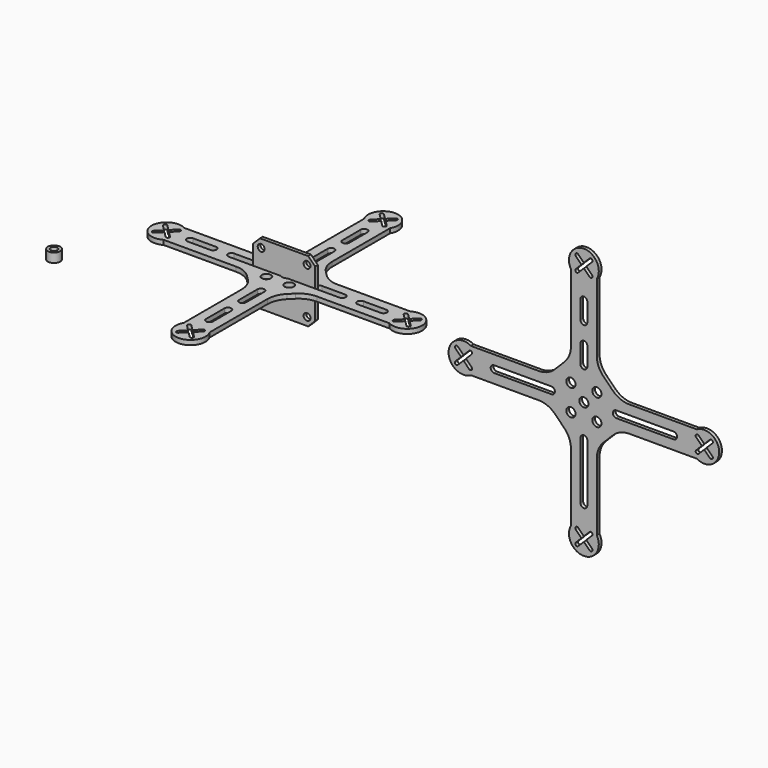
from build123d import *

# Parameters (mm, degrees)
F0_R     = 1.5
F1_DEPTH = 1.5
F0_R_2   = 2
F2_R     = 2
F3_DEPTH = 2
F2_R_2   = 2.7
F2_R_3   = 1.5
F4_DEPTH = 4


# Not quite as in the source:
# - ends of sketch curves that miss each other by under 0.0002 mm in the source are joined


with BuildPart() as f1:
    # F0 (on Front) → F1 (new body)
    with BuildSketch(Plane.XZ):
        Polygon((-10.5, 13.5), (-13.5, 10.5), (-13.5, -10.5), (-10.5, -13.5), (10.5, -13.5), (13.5, -10.5), (13.5, 10.5), (10.5, 13.5), align=None)
        with Locations((-10, -10)):
            Circle(F0_R, mode=Mode.SUBTRACT)
        with Locations((10, -10)):
            Circle(F0_R, mode=Mode.SUBTRACT)
        with Locations((-10, 10)):
            Circle(F0_R, mode=Mode.SUBTRACT)
        with Locations((10, 10)):
            Circle(F0_R, mode=Mode.SUBTRACT)
    extrude(amount=F1_DEPTH)


with BuildPart() as f1b:
    # F0 (on Front) → F1, piece 2 (new body)
    with BuildSketch(Plane.XZ):
        with BuildLine():
            Line((136.3622312263, 16.1907973599), (136.3622859694, 45.7145852416))
            ThreePointArc((136.3622859694, 45.7145852416), (130.7331330901, 55.4645956457), (125.1039619394, 45.7145956457))
            Line((125.1039619394, 45.7145956457), (125.1039619394, 16.1907616237))
            ThreePointArc((125.1039619394, 16.1907616237), (124.3427630001, 12.3639411471), (122.1750509474, 9.119715008))
            Line((122.1750509474, 9.119715008), (118.078023297, 5.0226627951))
            ThreePointArc((118.078023297, 5.0226627951), (114.8337738944, 2.8549162734), (111.006915747, 2.0937094108))
            Line((111.006915747, 2.0937094108), (81.4831278653, 2.0937641538))
            ThreePointArc((81.4831278653, 2.0937641538), (71.7331174612, -3.5353887254), (81.4831174612, -9.1645598762))
            Line((81.4831174612, -9.1645598762), (111.0069514832, -9.1645598762))
            ThreePointArc((111.0069514832, -9.1645598762), (114.8337719598, -9.9257588154), (118.0779980988, -12.0934708681))
            Line((118.0779980988, -12.0934708681), (122.1750503117, -16.1904985185))
            ThreePointArc((122.1750503117, -16.1904985185), (124.3427968334, -19.4347479211), (125.1040036961, -23.2616060685))
            Line((125.1040036961, -23.2616060685), (125.1039489531, -52.7853939503))
            ThreePointArc((125.1039489531, -52.7853939503), (130.7331018323, -62.5354043543), (136.362272983, -52.7854043543))
            Line((136.362272983, -52.7854043543), (136.362272983, -23.2615703324))
            ThreePointArc((136.362272983, -23.2615703324), (137.1234719223, -19.4347498558), (139.291183975, -16.1905237167))
            Line((139.291183975, -16.1905237167), (143.3882116254, -12.0934715038))
            ThreePointArc((143.3882116254, -12.0934715038), (146.632461028, -9.9257249821), (150.4593191754, -9.1645181195))
            Line((150.4593191754, -9.1645181195), (179.9831070571, -9.1645728625))
            ThreePointArc((179.9831070571, -9.1645728625), (189.7331174612, -3.5354199833), (179.9831174612, 2.0937511675))
            Line((179.9831174612, 2.0937511675), (150.4592834392, 2.0937511675))
            ThreePointArc((150.4592834392, 2.0937511675), (146.6324629627, 2.8549501067), (143.3882368236, 5.0226621595))
            Line((143.3882368236, 5.0226621595), (139.2911846107, 9.1196898098))
            ThreePointArc((139.2911846107, 9.1196898098), (137.123438089, 12.3639392124), (136.3622312263, 16.1907973599))
        make_face()
        with BuildLine():
            Line((116.5909818375, -5.0354043543), (91.5909818375, -5.0354043543))
            ThreePointArc((91.5909818375, -5.0354043543), (90.0909818375, -3.5354043543), (91.5909818375, -2.0354043543))
            Line((91.5909818375, -2.0354043543), (116.5909818375, -2.0354043543))
            ThreePointArc((116.5909818375, -2.0354043543), (118.0909818375, -3.5354043543), (116.5909818375, -5.0354043543))
        make_face(mode=Mode.SUBTRACT)
        with BuildLine():
            ThreePointArc((134.2686417644, -58.5102780885), (134.2686417644, -59.5709382603), (133.2079815926, -59.5709382603))
            Line((133.2079815926, -59.5709382603), (130.7318815655, -57.0948382332))
            Line((130.7318815655, -57.0948382332), (128.3029594878, -59.5220759616))
            ThreePointArc((128.3029594878, -59.5220759616), (127.2215110847, -59.593840654), (127.1975739525, -58.5102780885))
            Line((127.1975739844, -58.5102781204), (129.6724477185, -56.0354043862))
            Line((129.6724477185, -56.0354043862), (127.1975739525, -53.5605306202))
            ThreePointArc((127.1975739525, -53.5605306202), (127.1975739525, -52.4998704484), (128.2582341243, -52.4998704484))
            Line((128.2582341243, -52.4998704484), (130.7331078903, -54.9747442145))
            Line((130.7331078903, -54.9747442145), (133.2079816245, -52.4998704803))
            ThreePointArc((133.2079816245, -52.4998704803), (134.2686417325, -52.4998704803), (134.2686417325, -53.5605305883))
            Line((134.2686417644, -53.5605306202), (134.2684577566, -53.5607145003))
            Line((134.2684577566, -53.5607145003), (131.7929096252, -56.0345459493))
            Line((131.7929096252, -56.0345459493), (134.2686417644, -58.5102780885))
        make_face(mode=Mode.SUBTRACT)
        with BuildLine():
            Line((132.2331174612, -17.6775399781), (132.2331174612, -42.6775399781))
            ThreePointArc((132.2331174612, -42.6775399781), (130.7331174612, -44.1775399781), (129.2331174612, -42.6775399781))
            Line((129.2331174612, -42.6775399781), (129.2331174612, -17.6775399781))
            ThreePointArc((129.2331174612, -17.6775399781), (130.7331174612, -16.1775399781), (132.2331174612, -17.6775399781))
        make_face(mode=Mode.SUBTRACT)
        with Locations((125.0762632117, -9.1922586038)):
            Circle(F0_R_2, mode=Mode.SUBTRACT)
        with Locations((136.3899717107, -9.1922586038)):
            Circle(F0_R_2, mode=Mode.SUBTRACT)
        with Locations((130.7331174612, -3.5354043543)):
            Circle(F0_R_2, mode=Mode.SUBTRACT)
        with BuildLine():
            ThreePointArc((185.7079911954, 0.0001199488), (186.7686513671, 0.0001199488), (186.7686513671, -1.060540223))
            Line((186.7686513671, -1.060540223), (184.2925513401, -3.53664025))
            Line((184.2925513401, -3.53664025), (186.7197890684, -5.9655623277))
            ThreePointArc((186.7197890684, -5.9655623277), (186.7915537608, -7.0470107308), (185.7079911954, -7.070947863))
            Line((185.7079912273, -7.0709478311), (183.2331174931, -4.596074097))
            Line((183.2331174931, -4.596074097), (180.7582437271, -7.070947863))
            ThreePointArc((180.7582437271, -7.070947863), (179.6975835553, -7.070947863), (179.6975835553, -6.0102876913))
            Line((179.6975835553, -6.0102876913), (182.1724573213, -3.5354139252))
            Line((182.1724573213, -3.5354139252), (179.6975835872, -1.0605401911))
            ThreePointArc((179.6975835872, -1.0605401911), (179.6975835872, 0.0001199169), (180.7582436952, 0.0001199169))
            Line((180.7582437271, 0.0001199488), (180.7584276072, -6.40589e-05))
            Line((180.7584276072, -6.40589e-05), (183.2322590562, -2.4756121904))
            Line((183.2322590562, -2.4756121904), (185.7079911954, 0.0001199488))
        make_face(mode=Mode.SUBTRACT)
        with BuildLine():
            ThreePointArc((75.7582437271, -7.0709286575), (74.6975835553, -7.0709286575), (74.6975835553, -6.0102684857))
            Line((74.6975835553, -6.0102684857), (77.1736835823, -3.5341684586))
            Line((77.1736835823, -3.5341684586), (74.746445854, -1.1052463809))
            ThreePointArc((74.746445854, -1.1052463809), (74.6746811616, -0.0237979778), (75.7582437271, 0.0001391544))
            Line((75.7582436952, 0.0001391225), (78.2331174293, -2.4747346117))
            Line((78.2331174293, -2.4747346117), (80.7079911954, 0.0001391544))
            ThreePointArc((80.7079911954, 0.0001391544), (81.7686513671, 0.0001391544), (81.7686513671, -1.0605210174))
            Line((81.7686513671, -1.0605210174), (79.2937776011, -3.5353947835))
            Line((79.2937776011, -3.5353947835), (81.7686513352, -6.0102685176))
            ThreePointArc((81.7686513352, -6.0102685176), (81.7686513352, -7.0709286256), (80.7079912273, -7.0709286256))
            Line((80.7079911954, -7.0709286575), (80.7078073152, -7.0707446498))
            Line((80.7078073152, -7.0707446498), (78.2339758662, -4.5951965183))
            Line((78.2339758662, -4.5951965183), (75.7582437271, -7.0709286575))
        make_face(mode=Mode.SUBTRACT)
        with Locations((125.0762632117, 2.1214498952)):
            Circle(F0_R_2, mode=Mode.SUBTRACT)
        with Locations((136.3899717107, 2.1214498952)):
            Circle(F0_R_2, mode=Mode.SUBTRACT)
        with BuildLine():
            Line((144.8752530849, -2.0354043543), (169.8752530849, -2.0354043543))
            ThreePointArc((169.8752530849, -2.0354043543), (171.3752530849, -3.5354043543), (169.8752530849, -5.0354043543))
            Line((169.8752530849, -5.0354043543), (144.8752530849, -5.0354043543))
            ThreePointArc((144.8752530849, -5.0354043543), (143.3752530849, -3.5354043543), (144.8752530849, -2.0354043543))
        make_face(mode=Mode.SUBTRACT)
        with BuildLine():
            Line((132.2331174612, 18.6067312694), (132.2331174612, 10.6067312694))
            ThreePointArc((132.2331174612, 10.6067312694), (130.7331174612, 9.1067312694), (129.2331174612, 10.6067312694))
            Line((129.2331174612, 10.6067312694), (129.2331174612, 18.6067312694))
            ThreePointArc((129.2331174612, 18.6067312694), (130.7331174612, 20.1067312694), (132.2331174612, 18.6067312694))
        make_face(mode=Mode.SUBTRACT)
        with BuildLine():
            ThreePointArc((129.2331174612, 35.6067312694), (130.7331174612, 37.1067312694), (132.2331174612, 35.6067312694))
            Line((132.2331174612, 35.6067312694), (132.2331174612, 27.6067312694))
            ThreePointArc((132.2331174612, 27.6067312694), (130.7331174612, 26.1067312694), (129.2331174612, 27.6067312694))
            Line((129.2331174612, 27.6067312694), (129.2331174612, 35.6067312694))
        make_face(mode=Mode.SUBTRACT)
        with BuildLine():
            ThreePointArc((127.1975931581, 51.4394693798), (127.1975931581, 52.5001295516), (128.2582533298, 52.5001295516))
            Line((128.2582533298, 52.5001295516), (130.7343533569, 50.0240295245))
            Line((130.7343533569, 50.0240295245), (133.1632754346, 52.4512672529))
            ThreePointArc((133.1632754346, 52.4512672529), (134.2447238377, 52.5230319453), (134.2686609699, 51.4394693798))
            Line((134.268660938, 51.4394694117), (131.7937872039, 48.9645956776))
            Line((131.7937872039, 48.9645956776), (134.2686609699, 46.4897219115))
            ThreePointArc((134.2686609699, 46.4897219115), (134.2686609699, 45.4290617397), (133.2080007981, 45.4290617397))
            Line((133.2080007981, 45.4290617397), (130.7331270321, 47.9039355058))
            Line((130.7331270321, 47.9039355058), (128.2582532979, 45.4290617716))
            ThreePointArc((128.2582532979, 45.4290617716), (127.19759319, 45.4290617716), (127.19759319, 46.4897218796))
            Line((127.1975931581, 46.4897219115), (127.1977771658, 46.4899057916))
            Line((127.1977771658, 46.4899057916), (129.6733252972, 48.9637372406))
            Line((129.6733252972, 48.9637372406), (127.1975931581, 51.4394693798))
        make_face(mode=Mode.SUBTRACT)
    extrude(amount=F1_DEPTH)


with BuildPart() as f3:
    # F2 (on Top) → F3 (new body)
    with BuildSketch(Plane.XY):
        with BuildLine():
            ThreePointArc((5.6291651246, 49.25), (0, 59), (-5.6291651246, 49.25))
            Line((-5.6291651246, 49.25), (-5.6291651246, 17.6048535912))
            ThreePointArc((-5.6291651246, 17.6048535912), (-6.3903697995, 13.7780192675), (-8.5580973127, 10.5337857793))
            Line((-8.5580973127, 10.5337857793), (-10.5337857793, 8.5580973127))
            ThreePointArc((-10.5337857793, 8.5580973127), (-13.7780192675, 6.3903697995), (-17.6048535912, 5.6291651246))
            Line((-17.6048535912, 5.6291651246), (-49.25, 5.6291651246))
            ThreePointArc((-49.25, 5.6291651246), (-59, 0), (-49.25, -5.6291651246))
            Line((-49.25, -5.6291651246), (-17.6048535912, -5.6291651246))
            ThreePointArc((-17.6048535912, -5.6291651246), (-13.7780192675, -6.3903697995), (-10.5337857793, -8.5580973127))
            Line((-10.5337857793, -8.5580973127), (-8.5580973127, -10.5337857793))
            ThreePointArc((-8.5580973127, -10.5337857793), (-6.3903697995, -13.7780192675), (-5.6291651246, -17.6048535912))
            Line((-5.6291651246, -17.6048535912), (-5.6291651246, -49.25))
            ThreePointArc((-5.6291651246, -49.25), (0, -59), (5.6291651246, -49.25))
            Line((5.6291651246, -49.25), (5.6291651246, -17.6048535912))
            ThreePointArc((5.6291651246, -17.6048535912), (6.3903697995, -13.7780192675), (8.5580973127, -10.5337857793))
            Line((8.5580973127, -10.5337857793), (10.5337857793, -8.5580973127))
            ThreePointArc((10.5337857793, -8.5580973127), (13.7780192675, -6.3903697995), (17.6048535912, -5.6291651246))
            Line((17.6048535912, -5.6291651246), (49.25, -5.6291651246))
            ThreePointArc((49.25, -5.6291651246), (59, 0), (49.25, 5.6291651246))
            Line((49.25, 5.6291651246), (17.6048535912, 5.6291651246))
            ThreePointArc((17.6048535912, 5.6291651246), (13.7780192675, 6.3903697995), (10.5337857793, 8.5580973127))
            Line((10.5337857793, 8.5580973127), (8.5580973127, 10.5337857793))
            ThreePointArc((8.5580973127, 10.5337857793), (6.3903697995, 13.7780192675), (5.6291651246, 17.6048535912))
            Line((5.6291651246, 17.6048535912), (5.6291651246, 49.25))
        make_face()
        with BuildLine():
            Line((1.0606601718, -52.5), (3.5355339059, -54.9748737342))
            ThreePointArc((3.5355339059, -54.9748737342), (3.5355339059, -56.0355339059), (2.4748737342, -56.0355339059))
            Line((2.4748737342, -56.0355339059), (0, -53.5606601718))
            Line((0, -53.5606601718), (-2.4748737342, -56.0355339059))
            ThreePointArc((-2.4748737342, -56.0355339059), (-3.5355339059, -56.0355339059), (-3.5355339059, -54.9748737342))
            Line((-3.5355339059, -54.9748737342), (-1.0606601718, -52.5))
            Line((-1.0606601718, -52.5), (-3.5355339059, -50.0251262658))
            ThreePointArc((-3.5355339059, -50.0251262658), (-3.5355339059, -48.9644660941), (-2.4748737342, -48.9644660941))
            Line((-2.4748737342, -48.9644660941), (0, -51.4393398282))
            Line((0, -51.4393398282), (2.4748737342, -48.9644660941))
            ThreePointArc((2.4748737342, -48.9644660941), (3.5355339059, -48.9644660941), (3.5355339059, -50.0251262658))
            Line((3.5355339059, -50.0251262658), (1.0606601718, -52.5))
        make_face(mode=Mode.SUBTRACT)
        with BuildLine():
            Line((1.5, -32.14214), (1.5, -42.14214))
            ThreePointArc((1.5, -42.14214), (0, -43.64214), (-1.5, -42.14214))
            Line((-1.5, -42.14214), (-1.5, -32.14214))
            ThreePointArc((-1.5, -32.14214), (0, -30.64214), (1.5, -32.14214))
        make_face(mode=Mode.SUBTRACT)
        with BuildLine():
            ThreePointArc((1.5, -24.14214), (0, -25.64214), (-1.5, -24.14214))
            Line((-1.5, -24.14214), (-1.5, -14.14214))
            ThreePointArc((-1.5, -14.14214), (0, -12.64214), (1.5, -14.14214))
            Line((1.5, -14.14214), (1.5, -24.14214))
        make_face(mode=Mode.SUBTRACT)
        with BuildLine():
            Line((-52.5, -1.0606601718), (-54.9748737342, -3.5355339059))
            ThreePointArc((-54.9748737342, -3.5355339059), (-56.0355339059, -3.5355339059), (-56.0355339059, -2.4748737342))
            Line((-56.0355339059, -2.4748737342), (-53.5606601718, 0))
            Line((-53.5606601718, 0), (-56.0355339059, 2.4748737342))
            ThreePointArc((-56.0355339059, 2.4748737342), (-56.0355339059, 3.5355339059), (-54.9748737342, 3.5355339059))
            Line((-54.9748737342, 3.5355339059), (-52.5, 1.0606601718))
            Line((-52.5, 1.0606601718), (-50.0251262658, 3.5355339059))
            ThreePointArc((-50.0251262658, 3.5355339059), (-48.9644660941, 3.5355339059), (-48.9644660941, 2.4748737342))
            Line((-48.9644660941, 2.4748737342), (-51.4393398282, 0))
            Line((-51.4393398282, 0), (-48.9644660941, -2.4748737342))
            ThreePointArc((-48.9644660941, -2.4748737342), (-48.9644660941, -3.5355339059), (-50.0251262658, -3.5355339059))
            Line((-50.0251262658, -3.5355339059), (-52.5, -1.0606601718))
        make_face(mode=Mode.SUBTRACT)
        with BuildLine():
            Line((-32.14214, -1.5), (-42.14214, -1.5))
            ThreePointArc((-42.14214, -1.5), (-43.64214, 0), (-42.14214, 1.5))
            Line((-42.14214, 1.5), (-32.14214, 1.5))
            ThreePointArc((-32.14214, 1.5), (-30.64214, 0), (-32.14214, -1.5))
        make_face(mode=Mode.SUBTRACT)
        with Locations((-4.9497474683, -4.9497474683)):
            Circle(F2_R, mode=Mode.SUBTRACT)
        with BuildLine():
            ThreePointArc((-24.14214, -1.5), (-25.64214, 0), (-24.14214, 1.5))
            Line((-24.14214, 1.5), (-14.14214, 1.5))
            ThreePointArc((-14.14214, 1.5), (-12.64214, 0), (-14.14214, -1.5))
            Line((-14.14214, -1.5), (-24.14214, -1.5))
        make_face(mode=Mode.SUBTRACT)
        Circle(F2_R, mode=Mode.SUBTRACT)
        with Locations((4.9497474683, -4.9497474683)):
            Circle(F2_R, mode=Mode.SUBTRACT)
        with BuildLine():
            ThreePointArc((24.14214, 1.5), (25.64214, 0), (24.14214, -1.5))
            Line((24.14214, -1.5), (14.14214, -1.5))
            ThreePointArc((14.14214, -1.5), (12.64214, 0), (14.14214, 1.5))
            Line((14.14214, 1.5), (24.14214, 1.5))
        make_face(mode=Mode.SUBTRACT)
        with BuildLine():
            Line((32.14214, 1.5), (42.14214, 1.5))
            ThreePointArc((42.14214, 1.5), (43.64214, 0), (42.14214, -1.5))
            Line((42.14214, -1.5), (32.14214, -1.5))
            ThreePointArc((32.14214, -1.5), (30.64214, 0), (32.14214, 1.5))
        make_face(mode=Mode.SUBTRACT)
        with BuildLine():
            Line((52.5, 1.0606601718), (54.9748737342, 3.5355339059))
            ThreePointArc((54.9748737342, 3.5355339059), (56.0355339059, 3.5355339059), (56.0355339059, 2.4748737342))
            Line((56.0355339059, 2.4748737342), (53.5606601718, 0))
            Line((53.5606601718, 0), (56.0355339059, -2.4748737342))
            ThreePointArc((56.0355339059, -2.4748737342), (56.0355339059, -3.5355339059), (54.9748737342, -3.5355339059))
            Line((54.9748737342, -3.5355339059), (52.5, -1.0606601718))
            Line((52.5, -1.0606601718), (50.0251262658, -3.5355339059))
            ThreePointArc((50.0251262658, -3.5355339059), (48.9644660941, -3.5355339059), (48.9644660941, -2.4748737342))
            Line((48.9644660941, -2.4748737342), (51.4393398282, 0))
            Line((51.4393398282, 0), (48.9644660941, 2.4748737342))
            ThreePointArc((48.9644660941, 2.4748737342), (48.9644660941, 3.5355339059), (50.0251262658, 3.5355339059))
            Line((50.0251262658, 3.5355339059), (52.5, 1.0606601718))
        make_face(mode=Mode.SUBTRACT)
        with Locations((-4.9497474683, 4.9497474683)):
            Circle(F2_R, mode=Mode.SUBTRACT)
        with Locations((4.9497474683, 4.9497474683)):
            Circle(F2_R, mode=Mode.SUBTRACT)
        with BuildLine():
            Line((-1.5, 14.14214), (-1.5, 24.14214))
            ThreePointArc((-1.5, 24.14214), (0, 25.64214), (1.5, 24.14214))
            Line((1.5, 24.14214), (1.5, 14.14214))
            ThreePointArc((1.5, 14.14214), (0, 12.64214), (-1.5, 14.14214))
        make_face(mode=Mode.SUBTRACT)
        with BuildLine():
            ThreePointArc((1.5, 32.14214), (0, 30.64214), (-1.5, 32.14214))
            Line((-1.5, 32.14214), (-1.5, 42.14214))
            ThreePointArc((-1.5, 42.14214), (0, 43.64214), (1.5, 42.14214))
            Line((1.5, 42.14214), (1.5, 32.14214))
        make_face(mode=Mode.SUBTRACT)
        with BuildLine():
            Line((-1.0606601718, 52.5), (-3.5355339059, 54.9748737342))
            ThreePointArc((-3.5355339059, 54.9748737342), (-3.5355339059, 56.0355339059), (-2.4748737342, 56.0355339059))
            Line((-2.4748737342, 56.0355339059), (0, 53.5606601718))
            Line((0, 53.5606601718), (2.4748737342, 56.0355339059))
            ThreePointArc((2.4748737342, 56.0355339059), (3.5355339059, 56.0355339059), (3.5355339059, 54.9748737342))
            Line((3.5355339059, 54.9748737342), (1.0606601718, 52.5))
            Line((1.0606601718, 52.5), (3.5355339059, 50.0251262658))
            ThreePointArc((3.5355339059, 50.0251262658), (3.5355339059, 48.9644660941), (2.4748737342, 48.9644660941))
            Line((2.4748737342, 48.9644660941), (0, 51.4393398282))
            Line((0, 51.4393398282), (-2.4748737342, 48.9644660941))
            ThreePointArc((-2.4748737342, 48.9644660941), (-3.5355339059, 48.9644660941), (-3.5355339059, 50.0251262658))
            Line((-3.5355339059, 50.0251262658), (-1.0606601718, 52.5))
        make_face(mode=Mode.SUBTRACT)
    extrude(amount=F3_DEPTH)


with BuildPart() as f4:
    # F2 (on Top) → F4 (new body)
    with BuildSketch(Plane.XY):
        with Locations((-71.7615187168, -37.2250303626)):
            Circle(F2_R_2)
        with Locations((-71.7615187168, -37.2250303626)):
            Circle(F2_R_3, mode=Mode.SUBTRACT)
    extrude(amount=F4_DEPTH)


solid = Compound([f1.part, f1b.part, f3.part, f4.part])
